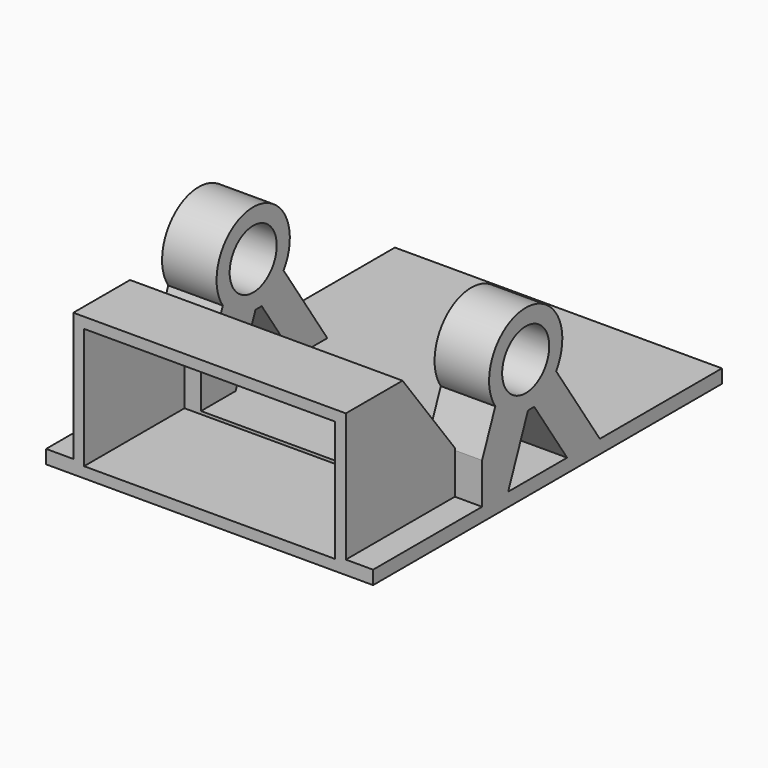
from build123d import *

# Parameters (mm, degrees)
F0_W          = 152.4
F0_H          = 203.2
F1_DEPTH      = 6.35
F3_DEPTH      = 63.5
F4_T          = 5
F4_T3_DEPTH   = 73.5
F4_T5_DEPTH   = 137
F6_R          = 13.716
F7_DEPTH      = 76.2
F5_W          = 101.6
F5_H          = 20
F8_DEPTH      = 63.501
F8_DEPTH_BACK = 139.701
F10_DEPTH     = 71.337


# Not quite as in the source:
# - a shell that OpenCascade refuses in one call is made with other operations: the cavity is built on its own and cut out


with BuildPart() as f1:
    # F0 (on Top) → F1 (new body)
    with BuildSketch(Plane.XY):
        Rectangle(F0_W, F0_H)
    extrude(amount=-F1_DEPTH)

    # F2 (on Right) → F3 (join, symmetric)
    with BuildSketch(Plane.YZ):
        Polygon((-101.6, 60), (-101.6, 0), (-38.1, 0), (-38.1, 20), (-68.58, 60), align=None)
    extrude(amount=F3_DEPTH, both=True)

    # F4: shell of thickness 5, made by hand


with BuildPart() as f4_core1:
    # F4_t2: copy of F1
    add(f1.part)

    # the walls: a layer under each face that stays
    f4_faces = [f4_core1.faces().sort_by_distance(p)[0] for p in [
        (0, 101.6, -3.175),
        (76.2, 0, -3.175),
        (-76.2, 0, -3.175),
        (0, 0, 0),
        (0, 0, -6.35),
        (63.5, -69.85, 30),
        (0, -38.1, 10),
        (-63.5, -69.85, 30),
        (0, -53.34, 40),
        (0, -85.09, 60),
    ]]
    thicken(f4_faces, amount=-F4_T, mode=Mode.SUBTRACT)

    # F4_s4 → F4_t3 (cut)
    with BuildSketch(Plane.XZ.offset(33.1)):
        Polygon((63.55, 0.05), (63.5, -5), (58.5, -5), (58.5, 0), align=None)
        Polygon((-63.55, 0.05), (-63.5, -5), (-58.5, -5), (-58.5, 0), align=None)
    extrude(amount=F4_T3_DEPTH, mode=Mode.SUBTRACT)

    # F4_s6 → F4_t5 (cut)
    with BuildSketch(Plane.YZ.offset(-68.5)):
        Polygon((-38.05, 0.05), (-38.1, -5), (-43.1, -5), (-43.1, 0), align=None)
    extrude(amount=F4_T5_DEPTH, mode=Mode.SUBTRACT)


with BuildPart() as f1_1:
    add(f1.part)

    # what is left inside the walls is the cavity
    f4_cavity = [f4_core1.part.solids().sort_by_distance(p)[0] for p in [
        (0, -82.1, -1.3),
    ]]
    add(f4_cavity, mode=Mode.SUBTRACT)

    # F6 (on Right) → F7 (join, symmetric)
    with BuildSketch(Plane.YZ):
        with BuildLine():
            Line((30.48, 0), (5.0091754749, 38.1))
            ThreePointArc((5.0091754749, 38.1), (-12.7, 71.336), (-30.4091754749, 38.1))
            Line((-30.4091754749, 38.1), (-38.1, 19.05))
            Line((-38.1, 19.05), (-38.1, 0))
            Line((-38.1, 0), (-22.9313431488, 0))
            Line((-22.9313431488, 0), (-11.3591754749, 28.664))
            Line((-11.3591754749, 28.664), (-7.7326171703, 28.664))
            Line((-7.7326171703, 28.664), (11.43, 0))
            Line((11.43, 0), (30.48, 0))
        make_face()
        with Locations((-12.7, 50)):
            Circle(F6_R, mode=Mode.SUBTRACT)
    extrude(amount=F7_DEPTH, both=True)

    # F5 (on face) → F8 (cut, two sides)
    with BuildSketch(Plane(origin=(0, -38.1, 0), x_dir=(-1, 0, 0), z_dir=(0, 1, 0))) as f8_sk:
        with Locations((0, 10)):
            Rectangle(F5_W, F5_H)
    extrude(amount=-F8_DEPTH, mode=Mode.SUBTRACT)
    extrude(f8_sk.sketch, amount=F8_DEPTH_BACK, mode=Mode.SUBTRACT)

    # F9 (on face) → F10 (cut, through all)
    with BuildSketch(Plane.XY):
        Polygon((50.8, 11.43), (50.8, 30.48), (-50.8, 30.48), (-50.8, 11.43), (-50.8, -22.9313431488), (-50.8, -38.1), (50.8, -38.1), (50.8, -22.9313431488), align=None)
    extrude(amount=F10_DEPTH, mode=Mode.SUBTRACT)


solid = f1_1.part
